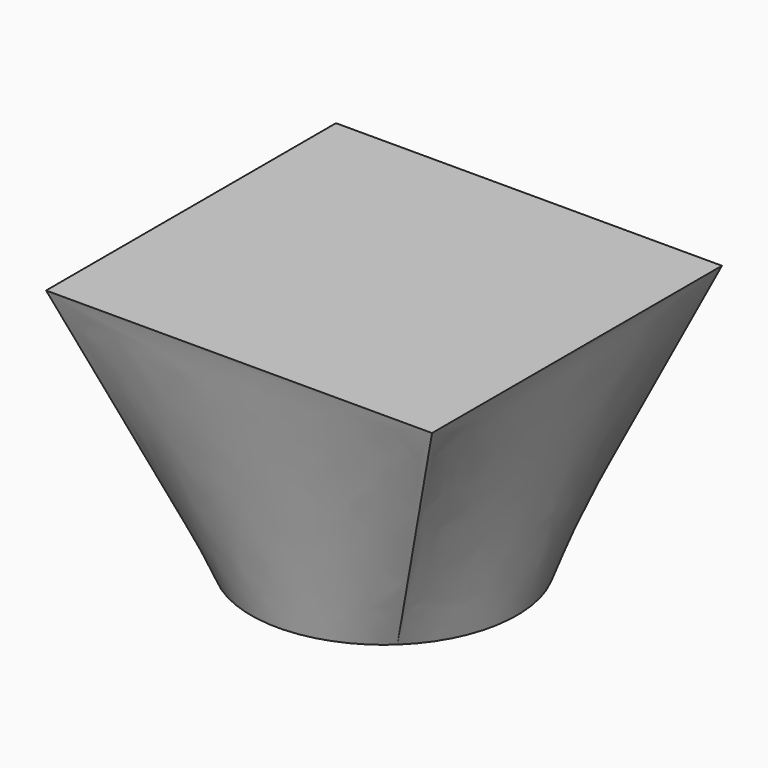
from build123d import *

# Parameters (mm, degrees)
F2_W = 77.3092359304
F2_H = 72.5790783763


# Not quite as in the source:
# - the arcs of a loft's sections are written as splines that run evenly, so that the points pair up as in the source's solid


with BuildPart() as f3:
    # F1 (on Top) → F3 section 0
    with BuildSketch(Plane.XY):
        with BuildLine():
            add(Edge.make_bspline(
                [(19.4270029416, 18.2383637886), (18.2333048231, 19.5098581578), (16.9144080528, 20.6637549911), (14.0767724731, 22.6921230133), (12.5581038297, 23.5665440468), (9.3792776513, 25.0023423072), (7.719198719, 25.5636840312), (4.3213424493, 26.3517356078), (2.5836491306, 26.5784259744), (-0.9026595196, 26.6884464872), (-2.6511886451, 26.5717739129), (-6.0919727893, 25.9995353351), (-7.7841427278, 25.5439834815), (-11.0471749612, 24.3114766208), (-12.617956571, 23.5345520901), (-15.5778403946, 21.6891414941), (-16.9668694194, 20.6207010602), (-18.2383637886, 19.4270029416)],
                knots=[0, 0, 0, 0, 0.125, 0.125, 0.25, 0.25, 0.375, 0.375, 0.5, 0.5, 0.625, 0.625, 0.75, 0.75, 0.875, 0.875, 1, 1, 1, 1], degree=3))
            add(Edge.make_bspline(
                [(-18.2383637886, 19.4270029416), (-19.5098581578, 18.2333048231), (-20.6637549911, 16.9144080528), (-22.6921230133, 14.0767724731), (-23.5665440468, 12.5581038297), (-25.0023423072, 9.3792776513), (-25.5636840312, 7.719198719), (-26.3517356078, 4.3213424493), (-26.5784259744, 2.5836491306), (-26.6884464872, -0.9026595196), (-26.5717739129, -2.6511886451), (-25.9995353351, -6.0919727893), (-25.5439834815, -7.7841427278), (-24.3114766208, -11.0471749612), (-23.5345520901, -12.617956571), (-21.6891414941, -15.5778403946), (-20.6207010602, -16.9668694194), (-19.4270029416, -18.2383637886)],
                knots=[0, 0, 0, 0, 0.125, 0.125, 0.25, 0.25, 0.375, 0.375, 0.5, 0.5, 0.625, 0.625, 0.75, 0.75, 0.875, 0.875, 1, 1, 1, 1], degree=3))
            add(Edge.make_bspline(
                [(-19.4270029416, -18.2383637886), (-18.2333048231, -19.5098581578), (-16.9144080528, -20.6637549911), (-14.0767724731, -22.6921230133), (-12.5581038297, -23.5665440468), (-9.3792776513, -25.0023423072), (-7.719198719, -25.5636840312), (-4.3213424493, -26.3517356078), (-2.5836491306, -26.5784259744), (0.9026595196, -26.6884464872), (2.6511886451, -26.5717739129), (6.0919727893, -25.9995353351), (7.7841427278, -25.5439834815), (11.0471749612, -24.3114766208), (12.617956571, -23.5345520901), (15.5778403946, -21.6891414941), (16.9668694194, -20.6207010602), (18.2383637886, -19.4270029416)],
                knots=[0, 0, 0, 0, 0.125, 0.125, 0.25, 0.25, 0.375, 0.375, 0.5, 0.5, 0.625, 0.625, 0.75, 0.75, 0.875, 0.875, 1, 1, 1, 1], degree=3))
            add(Edge.make_bspline(
                [(18.2383637886, -19.4270029416), (19.5098581578, -18.2333048231), (20.6637549911, -16.9144080528), (22.6921230133, -14.0767724731), (23.5665440468, -12.5581038297), (25.0023423072, -9.3792776513), (25.5636840312, -7.719198719), (26.3517356078, -4.3213424493), (26.5784259744, -2.5836491306), (26.6884464872, 0.9026595196), (26.5717739129, 2.6511886451), (25.9995353351, 6.0919727893), (25.5439834815, 7.7841427278), (24.3114766208, 11.0471749612), (23.5345520901, 12.617956571), (21.6891414941, 15.5778403946), (20.6207010602, 16.9668694194), (19.4270029416, 18.2383637886)],
                knots=[0, 0, 0, 0, 0.125, 0.125, 0.25, 0.25, 0.375, 0.375, 0.5, 0.5, 0.625, 0.625, 0.75, 0.75, 0.875, 0.875, 1, 1, 1, 1], degree=3))
        make_face()
    # F2 (on offset) → F3 section 1
    with BuildSketch(Plane.XY.offset(50.8)):
        Rectangle(F2_W, F2_H)
    loft(ruled=True)


solid = f3.part
